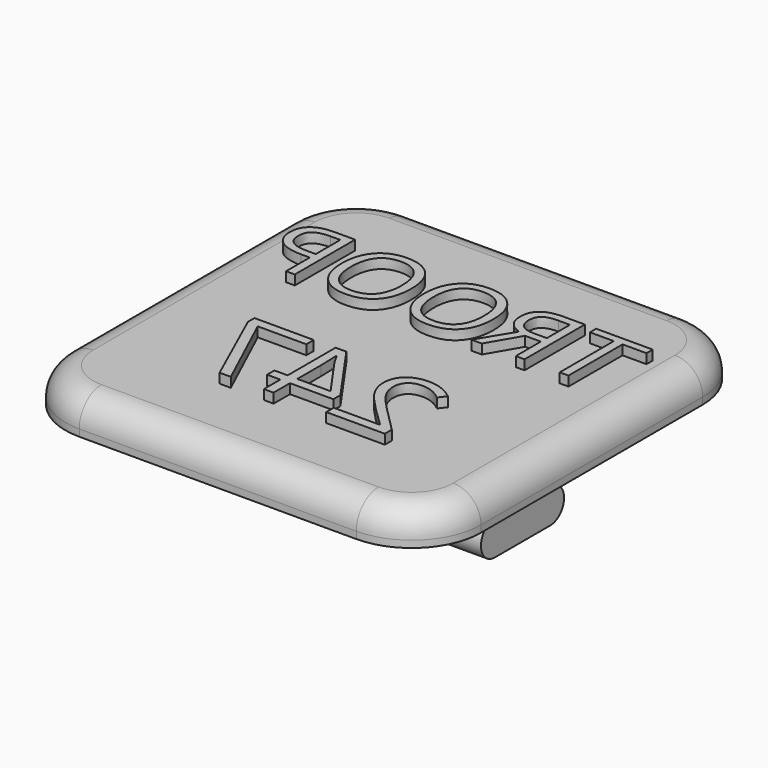
from build123d import *

# Parameters (mm, degrees)
F0_W           = 76.2
F0_H           = 76.2
F1_DEPTH       = 6.35
F2_R           = 12.7
F3_TEXT_SIZE   = 19.3616007623
F3_TEXT_SIZE_2 = 22.8914757792
F4_DEPTH       = 1.778
F5_R           = 5.08
F6_W           = 50.8
F6_H           = 12.7
F7_DEPTH       = 15.875
F9_DEPTH       = 50.8


# Not quite as in the source:
# - Text() gives the source's letters only with a copy of the font that has no kerning and outlines rounded to 1/6400 em; it was checked with that copy


with BuildPart() as f1:
    # F0 (on Top) → F1 (new body)
    with BuildSketch(Plane.XY):
        with Locations((38.1, -38.1)):
            Rectangle(F0_W, F0_H)
    extrude(amount=F1_DEPTH)

    # F2
    f2_edges = [f1.edges().sort_by_distance(p)[0] for p in [
        (0, -76.2, 3.175),
        (76.2, -76.2, 3.175),
        (76.2, 0, 3.175),
        (0, 0, 3.175),
    ]]
    fillet(f2_edges, radius=F2_R)

    # F3 (on face) → F4 (join)
    with BuildSketch(Plane.XY.offset(6.35)):
        with Locations((6.35, -29.8153525488)):
            Text('TROOP', F3_TEXT_SIZE, font='Open Sans', text_align=(TextAlign.LEFT, TextAlign.BOTTOM))
        with Locations((19.05, -60.325)):
            Text('247', F3_TEXT_SIZE_2, font='Open Sans', text_align=(TextAlign.LEFT, TextAlign.BOTTOM))
    extrude(amount=F4_DEPTH)

    # F5
    f5_edges = [f1.edges().sort_by_distance(p)[0] for p in [
        (3.719744, -72.480256, 6.35),
    ]]
    fillet(f5_edges, radius=F5_R)

    # F6 (on face) → F7 (join)
    with BuildSketch(Plane(origin=(0, 0, 0), x_dir=(1, 0, 0), z_dir=(0, 0, -1))):
        with Locations((38.1, 38.1)):
            Rectangle(F6_W, F6_H)
    extrude(amount=F7_DEPTH)

    # F8 (on face) → F9 (join, through all)
    with BuildSketch(Plane(origin=(12.7, 0, 0), x_dir=(0, -1, 0), z_dir=(-1, 0, 0))):
        with BuildLine():
            Line((44.45, -9.525), (44.45, -15.875))
            ThreePointArc((44.45, -15.875), (47.625, -12.7), (44.45, -9.525))
        make_face()
        with BuildLine():
            ThreePointArc((31.75, -9.525), (28.575, -12.7), (31.75, -15.875))
            Line((31.75, -15.875), (31.75, -9.525))
        make_face()
    extrude(amount=-F9_DEPTH)


with BuildPart() as f10_1:
    # F10: instance of F1
    add(f1.part.mirror(Plane.YZ))


solid = f10_1.part
